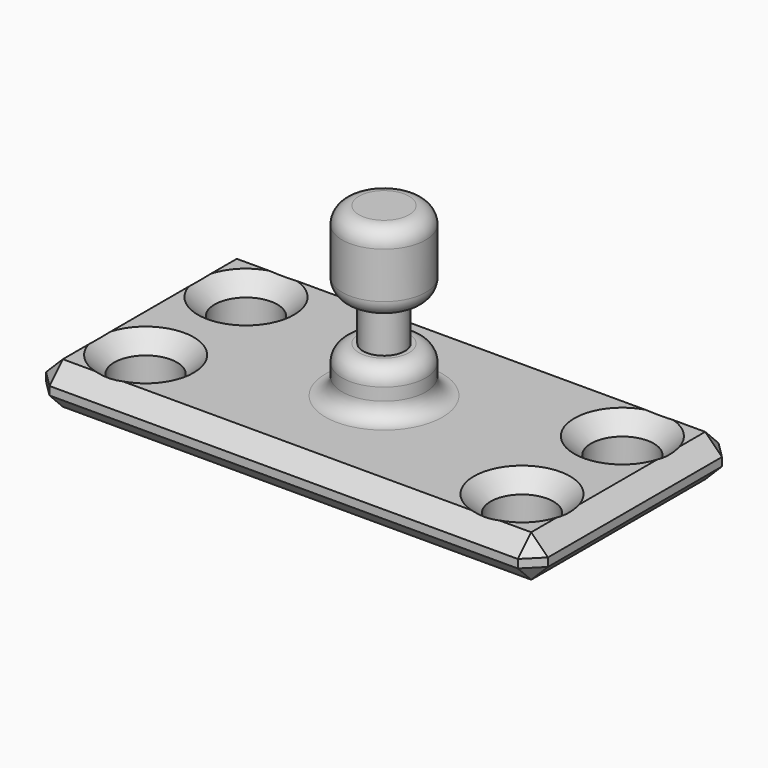
from build123d import *

# Parameters (mm, degrees)
F0_W         = 152.4
F0_H         = 76.2
F1_DEPTH     = 12.7
F2_R         = 9.525
F3_DEPTH     = 12.7
F4_W         = 12.7
F4_H         = 50.8
F6_W         = 7.62
F6_H         = 12.7
F8_R         = 5.08
F9_T1_DEPTH  = 6.4524666085
F9_T3_DEPTH  = 6.4524666085
F9_T5_DEPTH  = 6.4524666085
F9_T7_DEPTH  = 6.4524666085
F9_T9_DEPTH  = 6.4524666085
F9_T11_DEPTH = 6.4524666085
F9_T13_DEPTH = 6.4524666085
F9_T15_DEPTH = 6.4524666085
F9_T17_DEPTH = 102.3282991577
F9_T19_DEPTH = 178.5282991577
F9_T21_DEPTH = 38.8282991577


# Not quite as in the source:
# - a fillet or chamfer that OpenCascade refuses, or shapes differently, is made with other operations: its cross-section is extruded or revolved along the edge and cut away or added


with BuildPart() as f1:
    # F0 (on Top) → F1 (new body)
    with BuildSketch(Plane.XY):
        Rectangle(F0_W, F0_H)
    extrude(amount=F1_DEPTH)

    # F2 (on Top) → F3 (cut, symmetric)
    with BuildSketch(Plane.XY):
        with Locations((-57.15, 19.05)):
            Circle(F2_R)
        with Locations((57.15, 19.05)):
            Circle(F2_R)
        with Locations((57.15, -19.05)):
            Circle(F2_R)
        with Locations((-57.15, -19.05)):
            Circle(F2_R)
    extrude(amount=F3_DEPTH, both=True, mode=Mode.SUBTRACT)

    # F4 (on Front) → F5 (revolve)
    with BuildSketch(Plane.XZ):
        with Locations((6.35, 38.1)):
            Rectangle(F4_W, F4_H)
    revolve(axis=Axis((0, 0, 38.1), (0, 0, 1)))

    # F6 (on Front) → F7 (revolve, cut)
    with BuildSketch(Plane.XZ):
        with Locations((10.16, 32.980889082)):
            Rectangle(F6_W, F6_H)
    revolve(axis=Axis((0, 0, 12.7), (0, 0, 1)), mode=Mode.SUBTRACT)

    # F8
    f8_edges = [f1.edges().sort_by_distance(p)[0] for p in [
        (-12.7, 0, 12.7),
        (-12.7, 0, 63.5),
        (-12.7, 0, 26.630889),
        (-12.7, 0, 39.330889),
    ]]
    fillet(f8_edges, radius=F8_R)

    # F9: chamfer of 5.08 on 17 edges, made by hand

    # F9_s2 → F9_t1 (cut)
    with BuildSketch(Plane(origin=(38.9466666667, -38.9466666667, 38.9466666667), x_dir=(0.7071067812, 0.7071067812, 0), z_dir=(0.5773502692, -0.5773502692, 0.5773502692))):
        Polygon((26.9407683632, -32.1454703911), (30.5328708116, -38.3671743378), (23.3486659148, -38.3671743378), align=None)
    extrude(amount=F9_T1_DEPTH, mode=Mode.SUBTRACT)

    # F9_s4 → F9_t3 (cut)
    with BuildSketch(Plane(origin=(38.9466666667, 38.9466666667, 38.9466666667), x_dir=(-0.7071067812, 0.7071067812, 0), z_dir=(0.5773502692, 0.5773502692, 0.5773502692))):
        Polygon((-26.9407683632, -32.1454703911), (-30.5328708116, -38.3671743378), (-23.3486659148, -38.3671743378), align=None)
    extrude(amount=F9_T3_DEPTH, mode=Mode.SUBTRACT)

    # F9_s6 → F9_t5 (cut)
    with BuildSketch(Plane(origin=(-38.9466666667, -38.9466666667, 38.9466666667), x_dir=(0.7071067812, -0.7071067812, 0), z_dir=(-0.5773502692, -0.5773502692, 0.5773502692))):
        Polygon((-26.9407683632, -32.1454703911), (-23.3486659148, -38.3671743378), (-30.5328708116, -38.3671743378), align=None)
    extrude(amount=F9_T5_DEPTH, mode=Mode.SUBTRACT)

    # F9_s8 → F9_t7 (cut)
    with BuildSketch(Plane(origin=(-38.9466666667, 38.9466666667, 38.9466666667), x_dir=(-0.7071067812, -0.7071067812, 0), z_dir=(-0.5773502692, 0.5773502692, 0.5773502692))):
        Polygon((26.9407683632, -32.1454703911), (23.3486659148, -38.3671743378), (30.5328708116, -38.3671743378), align=None)
    extrude(amount=F9_T7_DEPTH, mode=Mode.SUBTRACT)

    # F9_s10 → F9_t9 (cut)
    with BuildSketch(Plane(origin=(-34.7133333333, -34.7133333333, -34.7133333333), x_dir=(0.7071067812, -0.7071067812, 0), z_dir=(-0.5773502692, -0.5773502692, -0.5773502692))):
        Polygon((-26.9407683632, 42.5149769689), (-23.3486659148, 48.7366809156), (-30.5328708116, 48.7366809156), align=None)
    extrude(amount=F9_T9_DEPTH, mode=Mode.SUBTRACT)

    # F9_s12 → F9_t11 (cut)
    with BuildSketch(Plane(origin=(34.7133333333, -34.7133333333, -34.7133333333), x_dir=(0.7071067812, 0.7071067812, 0), z_dir=(0.5773502692, -0.5773502692, -0.5773502692))):
        Polygon((26.9407683632, 42.5149769689), (30.5328708116, 48.7366809156), (23.3486659148, 48.7366809156), align=None)
    extrude(amount=F9_T11_DEPTH, mode=Mode.SUBTRACT)

    # F9_s14 → F9_t13 (cut)
    with BuildSketch(Plane(origin=(34.7133333333, 34.7133333333, -34.7133333333), x_dir=(-0.7071067812, 0.7071067812, 0), z_dir=(0.5773502692, 0.5773502692, -0.5773502692))):
        Polygon((-30.5328708116, 48.7366809156), (-26.9407683632, 42.5149769689), (-23.3486659148, 48.7366809156), align=None)
    extrude(amount=F9_T13_DEPTH, mode=Mode.SUBTRACT)

    # F9_s16 → F9_t15 (cut)
    with BuildSketch(Plane(origin=(-34.7133333333, 34.7133333333, -34.7133333333), x_dir=(-0.7071067812, -0.7071067812, 0), z_dir=(-0.5773502692, 0.5773502692, -0.5773502692))):
        Polygon((26.9407683632, 42.5149769689), (23.3486659148, 48.7366809156), (30.5328708116, 48.7366809156), align=None)
    extrude(amount=F9_T15_DEPTH, mode=Mode.SUBTRACT)

    # F9_s18 → F9_t17 (cut)
    with BuildSketch(Plane.XZ.offset(-51.1641495789)):
        Polygon((71.12, 12.7), (76.2, 7.62), (76.2, 12.7), align=None)
        Polygon((-71.12, 12.7), (-76.2, 7.62), (-76.2, 12.7), align=None)
        Polygon((-76.2, 5.08), (-71.12, 0), (-76.2, 0), align=None)
        Polygon((76.2, 5.08), (71.12, 0), (76.2, 0), align=None)
    extrude(amount=F9_T17_DEPTH, mode=Mode.SUBTRACT)

    # F9_s20 → F9_t19 (cut)
    with BuildSketch(Plane.YZ.offset(-89.2641495789)):
        Polygon((-33.02, 12.7), (-38.1, 7.62), (-38.1, 12.7), align=None)
        Polygon((33.02, 12.7), (38.1, 7.62), (38.1, 12.7), align=None)
        Polygon((-38.1, 5.08), (-33.02, 0), (-38.1, 0), align=None)
        Polygon((38.1, 5.08), (33.02, 0), (38.1, 0), align=None)
    extrude(amount=F9_T19_DEPTH, mode=Mode.SUBTRACT)

    # F9_s22 → F9_t21 (cut)
    with BuildSketch(Plane.XY.offset(-13.0641495789)):
        Polygon((-71.12, 38.1), (-76.2, 33.02), (-76.2, 38.1), align=None)
        Polygon((-71.12, -38.1), (-76.2, -33.02), (-76.2, -38.1), align=None)
        Polygon((76.2, -33.02), (71.12, -38.1), (76.2, -38.1), align=None)
        Polygon((76.2, 33.02), (71.12, 38.1), (76.2, 38.1), align=None)
    extrude(amount=F9_T21_DEPTH, mode=Mode.SUBTRACT)

    # F9_s23 → F9_t24 (revolve, cut)
    with BuildSketch(Plane.XZ.offset(19.05)):
        Polygon((-42.545, 12.7), (-47.625, 7.62), (-47.625, 12.7), align=None)
    revolve(axis=Axis((-57.15, -19.05, 12.7), (0, 0, 1)), mode=Mode.SUBTRACT)

    # F9_s25 → F9_t26 (revolve, cut)
    with BuildSketch(Plane.XZ.offset(19.05)):
        Polygon((71.755, 12.7), (66.675, 7.62), (66.675, 12.7), align=None)
    revolve(axis=Axis((57.15, -19.05, 12.7), (0, 0, 1)), mode=Mode.SUBTRACT)

    # F9_s27 → F9_t28 (revolve, cut)
    with BuildSketch(Plane.XZ.offset(-19.05)):
        Polygon((-42.545, 12.7), (-47.625, 7.62), (-47.625, 12.7), align=None)
    revolve(axis=Axis((-57.15, 19.05, 12.7), (0, 0, 1)), mode=Mode.SUBTRACT)

    # F9_s29 → F9_t30 (revolve, cut)
    with BuildSketch(Plane.XZ.offset(-19.05)):
        Polygon((71.755, 12.7), (66.675, 7.62), (66.675, 12.7), align=None)
    revolve(axis=Axis((57.15, 19.05, 12.7), (0, 0, 1)), mode=Mode.SUBTRACT)


solid = f1.part
